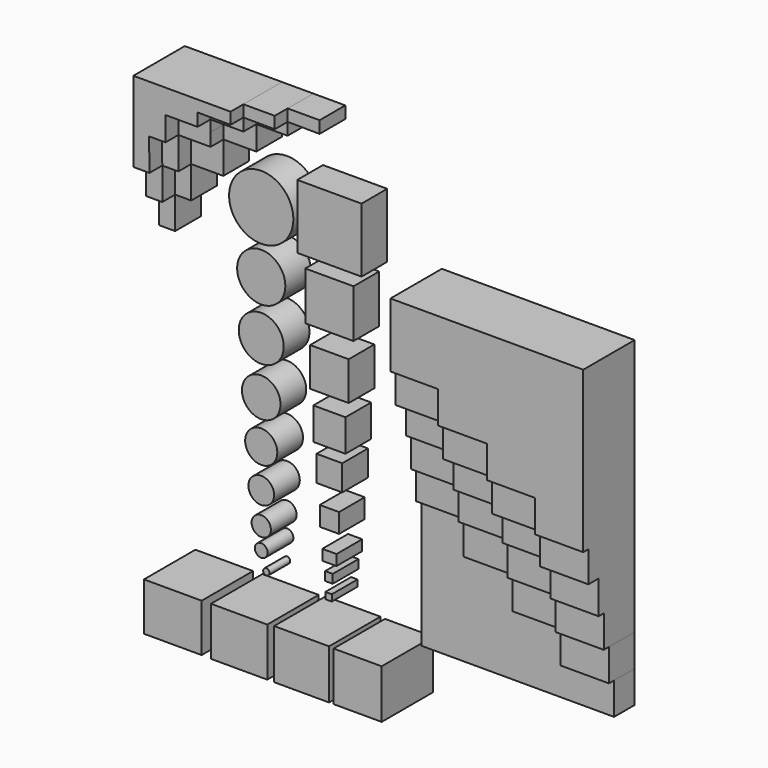
from build123d import *

# Parameters (mm, degrees)
F0_W      = 19.05
F0_H      = 12.7
F1_DEPTH  = 10.16
F0_R      = 1.27
F0_W_2    = 18.7868855402
F0_H_2    = 25.4
F2_DEPTH  = 25.4
F0_H_3    = 12.2142482221
F3_DEPTH  = 22.86
F0_H_4    = 13.1857517779
F4_DEPTH  = 17.78
F0_W_3    = 19.3131144598
F5_DEPTH  = 15.24
F6_DEPTH  = 12.7
F0_W_4    = 25.4
F7_DEPTH  = 12.7
F0_H_5    = 19.05
F0_W_5    = 15.24
F0_H_6    = 15.24
F0_W_6    = 12.7
F0_W_7    = 10.16
F0_H_7    = 10.16
F0_W_8    = 7.62
F0_H_8    = 7.62
F0_W_9    = 5.6200772524
F0_H_9    = 4.1779207373
F0_W_10   = 3.0056089163
F0_H_10   = 3.4552067518
F0_W_11   = 2.54
F0_H_11   = 2.54
F0_R_2    = 12.7
F8_DEPTH  = 12.7
F0_R_3    = 9.525
F0_R_4    = 8.89
F0_R_5    = 7.62
F0_R_6    = 6.35
F0_R_7    = 5.08
F0_R_8    = 3.81
F0_R_9    = 2.54
F0_W_12   = 22.7985456586
F0_H_12   = 18.9270973206
F10_DEPTH = 25.4
F0_W_13   = 22.2458466887
F0_H_13   = 19.1712155938
F11_DEPTH = 25.4
F0_W_14   = 21.7032656074
F0_H_14   = 19.5329338312
F12_DEPTH = 25.4
F0_W_15   = 18.9903564751
F0_H_15   = 19.3520784378
F13_DEPTH = 25.4
F0_W_16   = 6.3715364456
F0_H_16   = 4.4924213886
F0_W_17   = 6.3284635544
F0_H_17   = 5.0325786114
F14_DEPTH = 25.4
F0_W_18   = 6.35
F0_H_18   = 6.9809150934
F0_H_19   = 5.7190849066
F15_DEPTH = 12.7
F0_H_20   = 6.35
F0_H_21   = 7.1070512533
F0_H_22   = 5.5929487467
F16_DEPTH = 19.05
F0_H_23   = 5.0940299511
F0_H_24   = 4.4309700489


# Not quite as in the source:
# - the program builds the solid bodies; features that only make, move or delete a surface that nothing else refers to are left out


with BuildPart() as f1:
    # F0 (on Front) → F1 (new body)
    with BuildSketch(Plane.XZ):
        Polygon((-27.8272712708, -24.9142482221), (-27.8272712708, -76.2), (-9.0403857306, -76.2), (-9.0403857306, -38.1), (-9.0403857306, -24.9142482221), align=None)
        Polygon((-9.0403857306, -38.1), (-9.0403857306, -76.2), (10.2727287292, -76.2), (10.2727287292, -50.8), (10.2727287292, -38.1), align=None)
        Polygon((10.2727287292, -50.8), (10.2727287292, -76.2), (29.3227287292, -76.2), (29.3227287292, -63.5), (29.3227287292, -50.8), align=None)
        with Locations((38.8477287292, -69.85)):
            Rectangle(F0_W, F0_H)
    extrude(amount=F1_DEPTH)



with BuildPart() as f1b:
    # F0 (on Front) → F1, piece 2 (new body)
    with BuildSketch(Plane.XZ):
        with Locations((-89.0465825796, -70.4140141606)):
            Circle(F0_R)
    extrude(amount=F1_DEPTH)


with BuildPart() as f2:
    # F0 (on Front) → F2 (new body)
    with BuildSketch(Plane.XZ):
        with Locations((-18.4338285007, 38.1)):
            Rectangle(F0_W_2, F0_H_2)
        Polygon((10.2727287292, 50.8), (-9.0403857306, 50.8), (-9.0403857306, 25.4), (-9.0403857306, 12.7), (10.2727287292, 12.7), align=None)
        Polygon((29.3227287292, 50.8), (10.2727287292, 50.8), (10.2727287292, 12.7), (10.2727287292, 0), (29.3227287292, 0), align=None)
        Polygon((29.3227287292, 0), (29.3227287292, -12.7), (48.3727287292, -12.7), (48.3727287292, 50.8), (29.3227287292, 50.8), align=None)
    extrude(amount=F2_DEPTH)

    # F0 (on Front) → F3 (join)
    with BuildSketch(Plane.XZ):
        with Locations((-18.4338285007, 19.05)):
            Rectangle(F0_W_2, F0_H)
        Polygon((-9.0403857306, 12.7), (-9.0403857306, 0), (-8.7772712708, 0), (10.2727287292, 0), (10.2727287292, 12.7), align=None)
        with Locations((19.7977287292, -6.35)):
            Rectangle(F0_W, F0_H)
        with Locations((38.8477287292, -18.8071241111)):
            Rectangle(F0_W, F0_H_3)
    extrude(amount=F3_DEPTH)

    # F0 (on Front) → F4 (join)
    with BuildSketch(Plane.XZ):
        with Locations((-18.4338285007, 6.35)):
            Rectangle(F0_W_2, F0_H)
        Polygon((-9.0403857306, 0), (-9.0403857306, -12.7), (10.2727287292, -12.7), (10.2727287292, 0), (-8.7772712708, 0), align=None)
        with Locations((19.7977287292, -18.8071241111)):
            Rectangle(F0_W, F0_H_3)
        with Locations((38.8477287292, -31.5071241111)):
            Rectangle(F0_W, F0_H_4)
    extrude(amount=F4_DEPTH)


with BuildPart() as f1_1:
    add(f1.part)

    add(f2.part)  # F5 merges F2
    # F0 (on Front) → F5 (join)
    with BuildSketch(Plane.XZ):
        with Locations((-18.4338285007, -6.35)):
            Rectangle(F0_W_2, F0_H)
        with Locations((0.6161714993, -18.8071241111)):
            Rectangle(F0_W_3, F0_H_3)
        with Locations((19.7977287292, -31.5071241111)):
            Rectangle(F0_W, F0_H_4)
        with Locations((38.8477287292, -44.45)):
            Rectangle(F0_W, F0_H)
    extrude(amount=F5_DEPTH)


with BuildPart() as f6:
    # F0 (on Front) → F6 (new body)
    with BuildSketch(Plane.XZ):
        with Locations((-18.4338285007, -18.8071241111)):
            Rectangle(F0_W_2, F0_H_3)
    extrude(amount=F6_DEPTH)


with BuildPart() as f6b:
    # F0 (on Front) → F6, piece 2 (new body)
    with BuildSketch(Plane.XZ):
        with Locations((0.6161714993, -31.5071241111)):
            Rectangle(F0_W_3, F0_H_4)
    extrude(amount=F6_DEPTH)


with BuildPart() as f6c:
    # F0 (on Front) → F6, piece 3 (new body)
    with BuildSketch(Plane.XZ):
        with Locations((19.7977287292, -44.45)):
            Rectangle(F0_W, F0_H)
    extrude(amount=F6_DEPTH)


with BuildPart() as f6d:
    # F0 (on Front) → F6, piece 4 (new body)
    with BuildSketch(Plane.XZ):
        with Locations((38.8477287292, -57.15)):
            Rectangle(F0_W, F0_H)
    extrude(amount=F6_DEPTH)


with BuildPart() as f7:
    # F0 (on Front) → F7 (new body)
    with BuildSketch(Plane.XZ):
        with Locations((-62.1086061001, 58.9192248881)):
            Rectangle(F0_W_4, F0_H_2)
    extrude(amount=F7_DEPTH)


with BuildPart() as f7b:
    # F0 (on Front) → F7, piece 2 (new body)
    with BuildSketch(Plane.XZ):
        with Locations((-62.1086061001, 32.3015004396)):
            Rectangle(F0_W, F0_H_5)
    extrude(amount=F7_DEPTH)


with BuildPart() as f7c:
    # F0 (on Front) → F7, piece 3 (new body)
    with BuildSketch(Plane.XZ):
        with Locations((-62.1086061001, 8.2002608106)):
            Rectangle(F0_W_5, F0_H_6)
    extrude(amount=F7_DEPTH)


with BuildPart() as f7d:
    # F0 (on Front) → F7, piece 4 (new body)
    with BuildSketch(Plane.XZ):
        with Locations((-62.1086061001, -11.1287795007)):
            Rectangle(F0_W_6, F0_H)
    extrude(amount=F7_DEPTH)


with BuildPart() as f7e:
    # F0 (on Front) → F7, piece 5 (new body)
    with BuildSketch(Plane.XZ):
        with Locations((-62.1086061001, -26.2704808265)):
            Rectangle(F0_W_7, F0_H_7)
    extrude(amount=F7_DEPTH)


with BuildPart() as f7f:
    # F0 (on Front) → F7, piece 6 (new body)
    with BuildSketch(Plane.XZ):
        with Locations((-62.1086061001, -42.3916205764)):
            Rectangle(F0_W_8, F0_H_8)
    extrude(amount=F7_DEPTH)


with BuildPart() as f7g:
    # F0 (on Front) → F7, piece 7 (new body)
    with BuildSketch(Plane.XZ):
        with Locations((-62.1086061001, -55.6043089521)):
            Rectangle(F0_W_9, F0_H_9)
    extrude(amount=F7_DEPTH)


with BuildPart() as f7h:
    # F0 (on Front) → F7, piece 8 (new body)
    with BuildSketch(Plane.XZ):
        with Locations((-62.2849538922, -62.6233518124)):
            Rectangle(F0_W_10, F0_H_10)
    extrude(amount=F7_DEPTH)


with BuildPart() as f7i:
    # F0 (on Front) → F7, piece 9 (new body)
    with BuildSketch(Plane.XZ):
        with Locations((-62.4306201935, -69.3829506636)):
            Rectangle(F0_W_11, F0_H_11)
    extrude(amount=F7_DEPTH)


with BuildPart() as f8:
    # F0 (on Front) → F8 (new body)
    with BuildSketch(Plane.XZ):
        with Locations((-89.0465825796, 57.4598126113)):
            Circle(F0_R_2)
    extrude(amount=F8_DEPTH)


with BuildPart() as f8b:
    # F0 (on Front) → F8, piece 2 (new body)
    with BuildSketch(Plane.XZ):
        with Locations((-89.0465825796, 33.1723019481)):
            Circle(F0_R_3)
    extrude(amount=F8_DEPTH)


with BuildPart() as f8c:
    # F0 (on Front) → F8, piece 3 (new body)
    with BuildSketch(Plane.XZ):
        with Locations((-89.0465825796, 11.8560590819)):
            Circle(F0_R_4)
    extrude(amount=F8_DEPTH)


with BuildPart() as f8d:
    # F0 (on Front) → F8, piece 4 (new body)
    with BuildSketch(Plane.XZ):
        with Locations((-89.0465825796, -8.6508957956)):
            Circle(F0_R_5)
    extrude(amount=F8_DEPTH)


with BuildPart() as f8e:
    # F0 (on Front) → F8, piece 5 (new body)
    with BuildSketch(Plane.XZ):
        with Locations((-89.0465825796, -25.8254144788)):
            Circle(F0_R_6)
    extrude(amount=F8_DEPTH)


with BuildPart() as f8f:
    # F0 (on Front) → F8, piece 6 (new body)
    with BuildSketch(Plane.XZ):
        with Locations((-89.0465825796, -41.0346301064)):
            Circle(F0_R_7)
    extrude(amount=F8_DEPTH)


with BuildPart() as f8g:
    # F0 (on Front) → F8, piece 7 (new body)
    with BuildSketch(Plane.XZ):
        with Locations((-89.0465825796, -53.469389677)):
            Circle(F0_R_8)
    extrude(amount=F8_DEPTH)


with BuildPart() as f8h:
    # F0 (on Front) → F8, piece 8 (new body)
    with BuildSketch(Plane.XZ):
        with Locations((-89.0465825796, -61.9417019188)):
            Circle(F0_R_9)
    extrude(amount=F8_DEPTH)


with BuildPart() as f10:
    # F0 (on Front) → F10 (new body)
    with BuildSketch(Plane.XZ):
        with Locations((-113.8334684074, -88.0742967129)):
            Rectangle(F0_W_12, F0_H_12)
    extrude(amount=F10_DEPTH)


with BuildPart() as f11:
    # F0 (on Front) → F11 (new body)
    with BuildSketch(Plane.XZ):
        with Locations((-87.625619024, -88.0642943084)):
            Rectangle(F0_W_13, F0_H_13)
    extrude(amount=F11_DEPTH)


with BuildPart() as f12:
    # F0 (on Front) → F12 (new body)
    with BuildSketch(Plane.XZ):
        with Locations((-62.938157469, -87.8834351897)):
            Rectangle(F0_W_14, F0_H_14)
    extrude(amount=F12_DEPTH)


with BuildPart() as f13:
    # F0 (on Front) → F13 (new body)
    with BuildSketch(Plane.XZ):
        with Locations((-40.7827403396, -87.9738628864)):
            Rectangle(F0_W_15, F0_H_15)
    extrude(amount=F13_DEPTH)


with BuildPart() as f14:
    # F0 (on Front) → F14 (new body)
    with BuildSketch(Plane.XZ):
        Polygon((-129.4272712708, 95.25), (-129.4272712708, 90.7575786114), (-123.1464154059, 90.7575786114), (-123.1308728456, 95.25), align=None)
        Polygon((-129.4272712708, 90.7575786114), (-129.4272712708, 85.725), (-123.1638267636, 85.725), (-123.1464154059, 90.7575786114), align=None)
        Polygon((-129.4272712708, 85.725), (-129.4272712708, 81.2940299511), (-123.1791567189, 81.2940299511), (-123.1638267636, 85.725), align=None)
        Polygon((-123.1967806816, 76.2), (-129.4272712708, 76.2), (-129.4272712708, 70.6070512533), (-123.1441499722, 70.6070512533), align=None)
        Polygon((-123.1441499722, 70.6070512533), (-129.4272712708, 70.6070512533), (-129.4272712708, 63.5), (-123.0772712708, 63.5), align=None)
        Polygon((-129.4272712708, 81.2940299511), (-129.4272712708, 76.2), (-123.1967806816, 76.2), (-123.1791567189, 81.2940299511), align=None)
        Polygon((-123.1308728456, 95.25), (-123.1464154059, 90.7575786114), (-116.7272712708, 90.7575786114), (-116.7272712708, 95.25), align=None)
        with Locations((-113.5415030479, 93.0037893057)):
            Rectangle(F0_W_16, F0_H_16)
        with Locations((-107.1915030479, 93.0037893057)):
            Rectangle(F0_W_17, F0_H_16)
        Polygon((-104.0272712708, 95.25), (-104.0272712708, 90.7575786114), (-97.9933291674, 90.7147406639), (-97.9933291674, 95.25), align=None)
        Polygon((-97.9933291674, 95.25), (-97.9933291674, 90.7147406639), (-90.9974202514, 90.665073237), (-90.9974202514, 95.25), align=None)
        with Locations((-107.1915030479, 88.2412893057)):
            Rectangle(F0_W_17, F0_H_17)
        with Locations((-113.5415030479, 88.2412893057)):
            Rectangle(F0_W_16, F0_H_17)
        Polygon((-123.1464154059, 90.7575786114), (-123.1638267636, 85.725), (-116.7272712708, 85.725), (-116.7272712708, 90.7575786114), align=None)
        Polygon((-123.1638267636, 85.725), (-123.1791567189, 81.2940299511), (-116.7272712708, 81.2940299511), (-116.7272712708, 85.725), align=None)
        Polygon((-123.1791567189, 81.2940299511), (-123.1967806816, 76.2), (-116.7272712708, 76.2), (-116.7272712708, 81.2940299511), align=None)
    extrude(amount=F14_DEPTH)


with BuildPart() as f15:
    # F0 (on Front) → F15 (new body)
    with BuildSketch(Plane.XZ):
        with Locations((-126.2522712708, 41.5904575467)):
            Rectangle(F0_W_18, F0_H_18)
        with Locations((-126.2522712708, 47.9404575467)):
            Rectangle(F0_W_18, F0_H_19)
    extrude(amount=F15_DEPTH)


with BuildPart() as f15b:
    # F0 (on Front) → F15, piece 2 (new body)
    with BuildSketch(Plane.XZ):
        with Locations((-119.9022712708, 53.975)):
            Rectangle(F0_W_18, F0_H_20)
        with Locations((-119.9022712708, 60.325)):
            Rectangle(F0_W_18, F0_H_20)
    extrude(amount=F15_DEPTH)


with BuildPart() as f15c:
    # F0 (on Front) → F15, piece 3 (new body)
    with BuildSketch(Plane.XZ):
        with Locations((-113.5415030479, 67.0535256267)):
            Rectangle(F0_W_16, F0_H_21)
        with Locations((-113.5415030479, 73.4035256267)):
            Rectangle(F0_W_16, F0_H_22)
        with Locations((-107.1915030479, 73.4035256267)):
            Rectangle(F0_W_17, F0_H_22)
        with Locations((-107.1915030479, 67.0535256267)):
            Rectangle(F0_W_17, F0_H_21)
    extrude(amount=F15_DEPTH)


with BuildPart() as f15d:
    # F0 (on Front) → F15, piece 4 (new body)
    with BuildSketch(Plane.XZ):
        Polygon((-104.0014555308, 81.2940299511), (-103.9717766678, 76.2), (-98.1412529945, 76.2), (-98.0624615017, 81.2734826417), align=None)
        Polygon((-98.0624615017, 81.2734826417), (-98.1412529945, 76.2), (-90.9974202514, 76.2), (-90.9974202514, 81.2732434626), (-97.9933291674, 81.2732434626), align=None)
        Polygon((-104.0272712708, 85.725), (-104.0014555308, 81.2940299511), (-98.0624615017, 81.2734826417), (-97.9933291674, 85.725), align=None)
        Polygon((-97.9933291674, 85.725), (-98.0624615017, 81.2734826417), (-97.9933291674, 81.2732434626), (-90.9974202514, 81.2732434626), (-90.9974202514, 85.725), align=None)
    extrude(amount=F15_DEPTH)


with BuildPart() as f15e:
    # F0 (on Front) → F15, piece 5 (new body)
    with BuildSketch(Plane.XZ):
        Polygon((-90.9974202514, 90.665073237), (-90.9974202514, 85.725), (-84.9264413118, 85.725), (-84.9264413118, 90.6219723467), align=None)
        Polygon((-84.9264413118, 90.6219723467), (-84.9264413118, 85.725), (-78.6272712708, 85.725), (-78.6272712708, 90.5772514146), align=None)
    extrude(amount=F15_DEPTH)


with BuildPart() as f15f:
    # F0 (on Front) → F15, piece 6 (new body)
    with BuildSketch(Plane.XZ):
        Polygon((-78.6272712708, 95.25), (-78.6272712708, 90.5772514146), (-72.5964605808, 90.5344356986), (-72.5964605808, 95.25), align=None)
        Polygon((-72.5964605808, 95.25), (-72.5964605808, 90.5344356986), (-65.9853294492, 90.4875), (-65.9853294492, 95.25), align=None)
    extrude(amount=F15_DEPTH)


with BuildPart() as f16:
    # F0 (on Front) → F16 (new body)
    with BuildSketch(Plane.XZ):
        with Locations((-126.2522712708, 53.975)):
            Rectangle(F0_W_18, F0_H_20)
        with Locations((-126.2522712708, 60.325)):
            Rectangle(F0_W_18, F0_H_20)
    extrude(amount=F16_DEPTH)


with BuildPart() as f16b:
    # F0 (on Front) → F16, piece 2 (new body)
    with BuildSketch(Plane.XZ):
        Polygon((-116.7272712708, 70.6070512533), (-123.1441499722, 70.6070512533), (-123.0772712708, 63.5), (-116.7272712708, 63.5), align=None)
        Polygon((-116.7272712708, 76.2), (-123.1967806816, 76.2), (-123.1441499722, 70.6070512533), (-116.7272712708, 70.6070512533), align=None)
    extrude(amount=F16_DEPTH)


with BuildPart() as f16c:
    # F0 (on Front) → F16, piece 3 (new body)
    with BuildSketch(Plane.XZ):
        with Locations((-113.5415030479, 78.7470149755)):
            Rectangle(F0_W_16, F0_H_23)
        Polygon((-110.3557348251, 81.2940299511), (-110.3557348251, 76.2), (-104.0272712708, 76.2), (-103.9717766678, 76.2), (-104.0014555308, 81.2940299511), align=None)
        with Locations((-113.5415030479, 83.5095149755)):
            Rectangle(F0_W_16, F0_H_24)
        Polygon((-110.3557348251, 85.725), (-110.3557348251, 81.2940299511), (-104.0014555308, 81.2940299511), (-104.0272712708, 85.725), align=None)
    extrude(amount=F16_DEPTH)


with BuildPart() as f16d:
    # F0 (on Front) → F16, piece 4 (new body)
    with BuildSketch(Plane.XZ):
        Polygon((-104.0272712708, 90.7575786114), (-104.0272712708, 85.725), (-97.9933291674, 85.725), (-97.9933291674, 90.7147406639), align=None)
        Polygon((-97.9933291674, 90.7147406639), (-97.9933291674, 85.725), (-90.9974202514, 85.725), (-90.9974202514, 90.665073237), align=None)
    extrude(amount=F16_DEPTH)


with BuildPart() as f16e:
    # F0 (on Front) → F16, piece 5 (new body)
    with BuildSketch(Plane.XZ):
        Polygon((-90.9974202514, 95.25), (-90.9974202514, 90.665073237), (-84.9264413118, 90.6219723467), (-84.9264413118, 95.25), align=None)
        Polygon((-84.9264413118, 95.25), (-84.9264413118, 90.6219723467), (-78.6272712708, 90.5772514146), (-78.6272712708, 95.25), align=None)
    extrude(amount=F16_DEPTH)


solid = Compound([f1b.part, f1_1.part, f6.part, f6b.part, f6c.part, f6d.part, f7.part, f7b.part, f7c.part, f7d.part, f7e.part, f7f.part, f7g.part, f7h.part, f7i.part, f8.part, f8b.part, f8c.part, f8d.part, f8e.part, f8f.part, f8g.part, f8h.part, f10.part, f11.part, f12.part, f13.part, f14.part, f15.part, f15b.part, f15c.part, f15d.part, f15e.part, f15f.part, f16.part, f16b.part, f16c.part, f16d.part, f16e.part])
